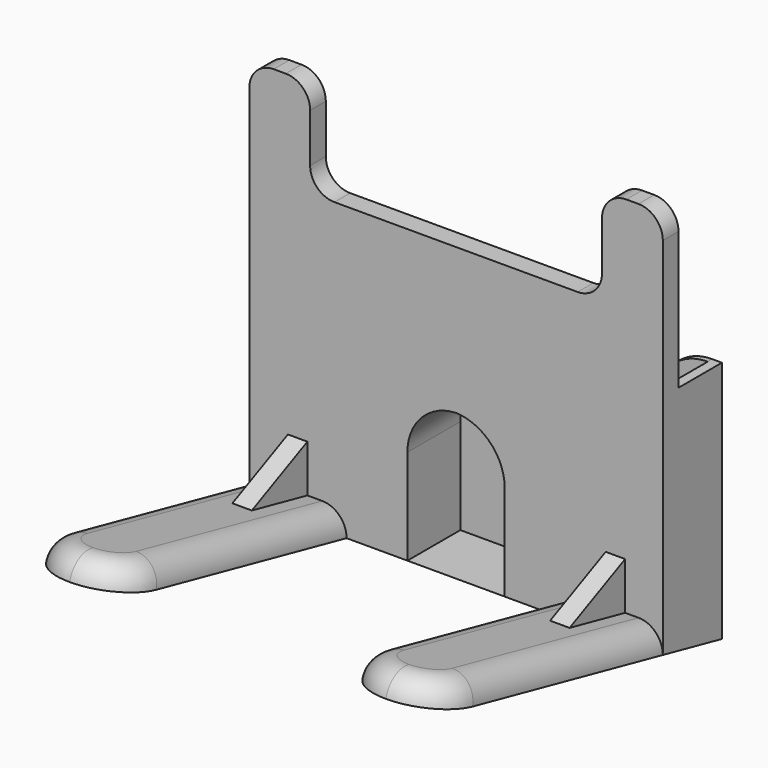
from build123d import *

# Parameters (mm, degrees)
F1_DEPTH      = 85
F3_W          = 81
F3_H          = 10
F4_DEPTH      = 20
F7_DEPTH      = 13.6
F9_W          = 60
F9_H          = 20
F10_DEPTH     = 2
F12_W         = 20
F12_H         = 60
F13_DEPTH     = 5
F14_T1_DEPTH  = 55
F15_R         = 4.99999
F16_R         = 10
F18_W         = 60
F18_H         = 20
F19_DEPTH     = 4.5
F20_R         = 5
F21_R         = 10.4535447251
F22_W         = 4
F22_H         = 13
F23_DEPTH     = 20
F24_T4_DEPTH  = 107.6390188569
F25_W         = 4
F25_H         = 9.7337032971
F26_DEPTH     = 15
F27_T4_DEPTH  = 81.7292641427
F28_T1_DEPTH  = 4.0324145269
F28_T6_DEPTH  = 55.9380061179
F28_T13_DEPTH = 55.9380061179
F28_T20_DEPTH = 29.9852103224
F28_T26_DEPTH = 55.9380061179


# Not quite as in the source:
# - a fillet or chamfer that OpenCascade refuses, or shapes differently, is made with other operations: its cross-section is extruded or revolved along the edge and cut away or added
# - a fillet or chamfer is up to 0.001 mm smaller than in the source, because OpenCascade refuses the exact size


with BuildPart() as f1:
    # F0 (on Right) → F1 (new body)
    with BuildSketch(Plane.YZ):
        Polygon((-12.1484044939, 63.271041885), (-12.1484044939, -16.728958115), (3.0366472241, -20.0031517962), (3.0366472241, 29.9968482038), (-8.115989967, 29.9968482038), (-8.115989967, 63.271041885), align=None)
    extrude(amount=F1_DEPTH)

    # F3 (on offset) → F4 (cut)
    with BuildSketch(Plane.XY.offset(30.2968482038)):
        with Locations((42.5, -3.115989967)):
            Rectangle(F3_W, F3_H)
    extrude(amount=-F4_DEPTH, mode=Mode.SUBTRACT)

    # F6 (on offset) → F7 (cut)
    with BuildSketch(Plane.XZ.offset(12.1484044939)):
        Polygon((32.5, -16.728958115), (42.5, -16.728958115), (52.5, -16.728958115), (52.5, 13.271041885), (42.5, 13.271041885), (32.5, 13.271041885), align=None)
    extrude(amount=-F7_DEPTH, mode=Mode.SUBTRACT)

    # F9 (on offset) → F10 (cut)
    with BuildSketch(Plane(origin=(0, 3.0366472241, 0), x_dir=(-1, 0, 0), z_dir=(0, 1, 0))):
        with Locations((-42.5, 19.9968482038)):
            Rectangle(F9_W, F9_H)
    extrude(amount=-F10_DEPTH, mode=Mode.SUBTRACT)

    # F12 (on offset) → F13 (join)
    with BuildSketch(Plane(origin=(0, -3.986549235, -18.488813492), x_dir=(1, 0, 0), z_dir=(0, -0.210775525, -0.9775344894))):
        with Locations((75, 38.3494294545)):
            Rectangle(F12_W, F12_H)
        with Locations((10, 38.3494294545)):
            Rectangle(F12_W, F12_H)
    extrude(amount=-F13_DEPTH)

    # F14: fillet of radius 10 on 4 edges, made by hand

    # F14_s2 → F14_t1 (cut)
    with BuildSketch(Plane(origin=(0, -9.2559373608, -42.927175728), x_dir=(1, 0, 0), z_dir=(0, 0.210775525, 0.9775344894))):
        with BuildLine():
            ThreePointArc((75, -68.3494294545), (67.9289321881, -65.4204972664), (65, -58.3494294545))
            Line((65, -58.3494294545), (65, -68.3494294545))
            Line((65, -68.3494294545), (75, -68.3494294545))
        make_face()
        with BuildLine():
            ThreePointArc((10, -68.3494294545), (2.9289321881, -65.4204972664), (0, -58.3494294545))
            Line((0, -58.3494294545), (0, -68.3494294545))
            Line((0, -68.3494294545), (10, -68.3494294545))
        make_face()
        with BuildLine():
            ThreePointArc((20, -58.3494294545), (17.0710678119, -65.4204972664), (10, -68.3494294545))
            Line((10, -68.3494294545), (20, -68.3494294545))
            Line((20, -68.3494294545), (20, -58.3494294545))
        make_face()
        with BuildLine():
            ThreePointArc((75, -68.3494294545), (82.0710678119, -65.4204972664), (85, -58.3494294545))
            Line((85, -58.3494294545), (85, -68.3494294545))
            Line((85, -68.3494294545), (75, -68.3494294545))
        make_face()
    extrude(amount=F14_T1_DEPTH, mode=Mode.SUBTRACT)

    # F15 (radius 5 in the source; OpenCascade refuses exactly that, so slightly less here)
    f15_edges = [f1.edges().sort_by_distance(p)[0] for p in [
        (85, -36.059828, -6.458279),
        (20, -36.059828, -6.458279),
    ]]
    fillet(f15_edges, radius=F15_R)

    # F16
    f16_edges = [f1.edges().sort_by_distance(p)[0] for p in [
        (12.5, 2.036647, 9.996848),
        (72.5, 2.036647, 9.996848),
    ]]
    fillet(f16_edges, radius=F16_R)

    # F18 (on offset) → F19 (cut)
    with BuildSketch(Plane(origin=(0, -8.115989967, 0), x_dir=(-1, 0, 0), z_dir=(0, 1, 0))):
        with Locations((-42.5, 53.271041885)):
            Rectangle(F18_W, F18_H)
    extrude(amount=-F19_DEPTH, mode=Mode.SUBTRACT)

    # F20
    f20_edges = [f1.edges().sort_by_distance(p)[0] for p in [
        (72.5, -10.132197, 63.271042),
        (85, -10.132197, 63.271042),
        (72.5, -10.132197, 43.271042),
        (12.5, -10.132197, 43.271042),
        (12.5, -10.132197, 63.271042),
        (0, -10.132197, 63.271042),
    ]]
    fillet(f20_edges, radius=F20_R)

    # F21
    f21_edges = [f1.edges().sort_by_distance(p)[0] for p in [
        (72.5, 2.460329, 29.996848),
        (12.5, 2.460329, 29.996848),
    ]]
    fillet(f21_edges, radius=F21_R)

    # F22 (on offset) → F23 (join)
    with BuildSketch(Plane(origin=(0, -8.115989967, 0), x_dir=(-1, 0, 0), z_dir=(0, 1, 0))):
        with Locations((-9.9369510557, -6.5)):
            Rectangle(F22_W, F22_H)
    extrude(amount=-F23_DEPTH)

    # F24: chamfer of 20 x 9.3261531631 on 1 edges, made by hand


with BuildPart() as f24_tool2:
    # F24_s3 → F24_t4 (new body)
    with BuildSketch(Plane.YZ.offset(-43.8825583727)):
        Polygon((-8.115989967, 0), (-28.115989967, -9.3261531631), (-28.115989967, 0), align=None)
    extrude(amount=F24_T4_DEPTH)

    split(bisect_by=Plane.XZ.offset(12.1484044939), keep=Keep.TOP)

    split(bisect_by=Plane(origin=(0, -2.9326716098, -13.6011410448), x_dir=(1, 0, 0), z_dir=(0, 0.210775525, 0.9775344894)), keep=Keep.TOP)


with BuildPart() as f1_1:
    add(f1.part)

    # F24_t1: cut F24_tool2
    add(f24_tool2.part, mode=Mode.SUBTRACT)

    # F25 (on face) → F26 (join)
    with BuildSketch(Plane.XZ.offset(12.1484044939)):
        with Locations((75.2541754842, -6.7471974233)):
            Rectangle(F25_W, F25_H)
    extrude(amount=F26_DEPTH)

    # F27: chamfer of 15 x 6.9946148723 on 1 edges, made by hand


with BuildPart() as f27_tool2:
    # F27_s3 → F27_t4 (new body)
    with BuildSketch(Plane.YZ.offset(116.1188075555)):
        Polygon((-12.1484044939, -1.8803457748), (-27.1484044939, -8.8749606471), (-27.1484044939, -1.8803457748), align=None)
    extrude(amount=-F27_T4_DEPTH)

    split(bisect_by=Plane.XZ.offset(12.1484044939), keep=Keep.TOP)

    split(bisect_by=Plane(origin=(0, -2.9326716098, -13.6011410448), x_dir=(1, 0, 0), z_dir=(0, 0.210775525, 0.9775344894)), keep=Keep.TOP)


with BuildPart() as f1_2:
    add(f1_1.part)

    # F27_t1: cut F27_tool2
    add(f27_tool2.part, mode=Mode.SUBTRACT)

    # F28: fillet of radius 10.3811183182 on 2 edges, made by hand

    # F28_s2 → F28_t1 (join)
    with BuildSketch(Plane.XZ.offset(8.115989967)):
        with BuildLine():
            ThreePointArc((42.8811183182, 13.271041885), (35.5405591591, 10.2304827259), (32.5, 2.8899235668))
            Line((32.5, 2.8899235668), (32.5, 13.271041885))
            Line((32.5, 13.271041885), (42.8811183182, 13.271041885))
        make_face()
        with BuildLine():
            ThreePointArc((52.5, 2.8899235668), (49.4594408409, 10.2304827259), (42.1188816818, 13.271041885))
            Line((42.1188816818, 13.271041885), (52.5, 13.271041885))
            Line((52.5, 13.271041885), (52.5, 2.8899235668))
        make_face()
    extrude(amount=F28_T1_DEPTH)


with BuildPart() as f28_tool4:
    # F28_s5 → F28_t6 (new body)
    with BuildSketch(Plane.XZ.offset(38.1012002894)):
        with BuildLine():
            ThreePointArc((42.8811183182, 13.271041885), (35.5405591591, 10.2304827259), (32.5, 2.8899235668))
            Line((32.5, 2.8899235668), (32.5, 13.271041885))
            Line((32.5, 13.271041885), (42.8811183182, 13.271041885))
        make_face()
    extrude(amount=-F28_T6_DEPTH)

    split(bisect_by=Plane.XZ.offset(-1.0366472241), keep=Keep.TOP)

    split(bisect_by=Plane.XY.offset(10.2968482038), keep=Keep.BOTTOM)

    split(bisect_by=Plane.XZ.offset(8.115989967), keep=Keep.BOTTOM)


with BuildPart() as f1_3:
    add(f1_2.part)

    # F28_t3: union F28_tool4
    add(f28_tool4.part)


with BuildPart() as f28_tool11:
    # F28_s12 → F28_t13 (new body)
    with BuildSketch(Plane.XZ.offset(38.1012002894)):
        with BuildLine():
            ThreePointArc((42.8811183182, 13.271041885), (35.5405591591, 10.2304827259), (32.5, 2.8899235668))
            Line((32.5, 2.8899235668), (32.5, 13.271041885))
            Line((32.5, 13.271041885), (42.8811183182, 13.271041885))
        make_face()
    extrude(amount=-F28_T13_DEPTH)

    split(bisect_by=Plane.XY.offset(9.9968482038), keep=Keep.BOTTOM)

    split(bisect_by=Plane.XZ.offset(8.115989967), keep=Keep.BOTTOM)

    split(bisect_by=Plane.XZ.offset(-3.0366472241), keep=Keep.TOP)


with BuildPart() as f1_4:
    add(f1_3.part)

    # F28_t10: union F28_tool11
    add(f28_tool11.part)


with BuildPart() as f28_tool18:
    # F28_s19 → F28_t20 (new body)
    with BuildSketch(Plane.XZ.offset(12.1484044939)):
        with BuildLine():
            ThreePointArc((52.5, 2.8899235668), (49.4594408409, 10.2304827259), (42.1188816818, 13.271041885))
            Line((42.1188816818, 13.271041885), (52.5, 13.271041885))
            Line((52.5, 13.271041885), (52.5, 2.8899235668))
        make_face()
    extrude(amount=-F28_T20_DEPTH)

    split(bisect_by=Plane.XY.offset(10.2968482038), keep=Keep.BOTTOM)

    split(bisect_by=Plane.XZ.offset(-1.0366472241), keep=Keep.TOP)


with BuildPart() as f1_5:
    add(f1_4.part)

    # F28_t17: union F28_tool18
    add(f28_tool18.part)


with BuildPart() as f28_tool24:
    # F28_s25 → F28_t26 (new body)
    with BuildSketch(Plane.XZ.offset(38.1012002894)):
        with BuildLine():
            ThreePointArc((52.5, 2.8899235668), (49.4594408409, 10.2304827259), (42.1188816818, 13.271041885))
            Line((42.1188816818, 13.271041885), (52.5, 13.271041885))
            Line((52.5, 13.271041885), (52.5, 2.8899235668))
        make_face()
    extrude(amount=-F28_T26_DEPTH)

    split(bisect_by=Plane.XY.offset(9.9968482038), keep=Keep.BOTTOM)

    split(bisect_by=Plane.XZ.offset(8.115989967), keep=Keep.BOTTOM)

    split(bisect_by=Plane.XZ.offset(-3.0366472241), keep=Keep.TOP)


with BuildPart() as f1_6:
    add(f1_5.part)

    # F28_t23: union F28_tool24
    add(f28_tool24.part)


solid = f1_6.part
